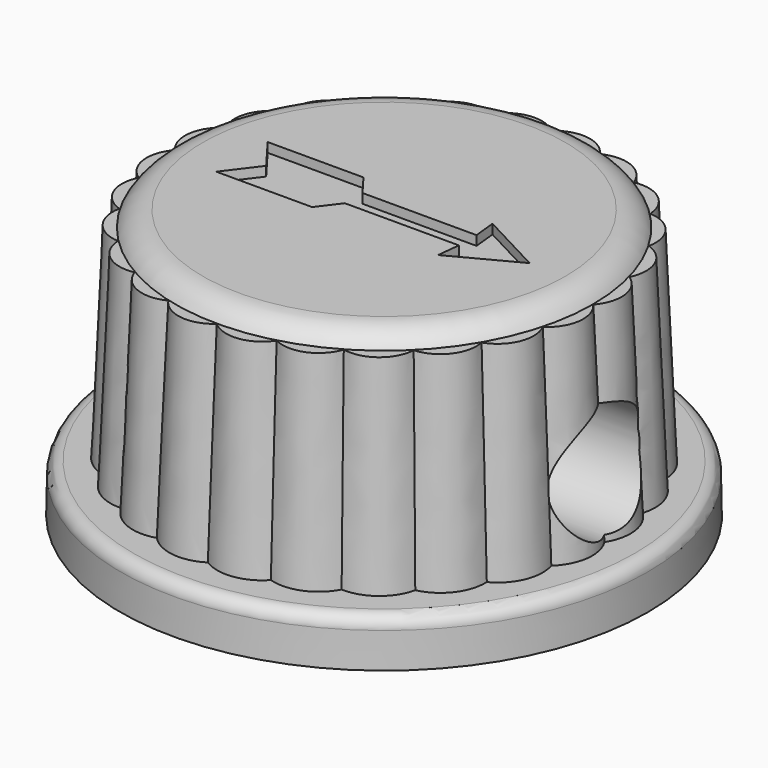
from build123d import *

# Parameters (mm, degrees)
F0_R                   = 8.35
F1_DEPTH               = 1.5
F1_TAPER               = 1
F2_R                   = 6.9
F3_DEPTH               = 6.5
F3_TAPER               = 2.5
F4_R                   = 6.6019829431
F5_DEPTH               = 0.5
F7_DEPTH               = 6.5
DRAFT_F7_DRAFTED_ANGLE = -2.5
F9_R                   = 0.4
F10_R                  = 3.9
F11_DEPTH              = 6.8
F12_R                  = 1.8
F13_DEPTH              = 25
F15_DEPTH              = 0.3


# Not quite as in the source:
# - a fillet or chamfer that OpenCascade refuses, or shapes differently, is made with other operations: its cross-section is extruded or revolved along the edge and cut away or added
# - an extrude with a draft is written as a straight extrude whose walls are then drafted


with BuildPart() as f1:
    # F0 (on Top) → F1 (new body)
    with BuildSketch(Plane.XY):
        Circle(F0_R)
    extrude(amount=F1_DEPTH, taper=F1_TAPER)

    # F2 (on face) → F3 (join)
    with BuildSketch(Plane.XY.offset(1.5)):
        Circle(F2_R)
    extrude(amount=F3_DEPTH, taper=F3_TAPER)

    # F4 (on face) → F5 (join)
    with BuildSketch(Plane.XY.offset(8)):
        Circle(F4_R)
    extrude(amount=F5_DEPTH)


with BuildPart() as f7_drafted:
    # F6 (on face) → F7 (new body, through all)
    with BuildSketch(Plane.XY.offset(8)):
        with BuildLine():
            ThreePointArc((6.3907621911, -1.7123995681), (6.8957390773, -0.9078412722), (6.6162038711, 0))
            ThreePointArc((6.6162038711, 0), (6.8957390773, 0.9078412722), (6.3907621911, 1.7123995681))
            ThreePointArc((6.3907621911, 1.7123995681), (6.4258058549, 2.6616559343), (5.729800629, 3.3081019355))
            ThreePointArc((5.729800629, 3.3081019355), (5.5179645827, 4.234083143), (4.678362623, 4.678362623))
            ThreePointArc((4.678362623, 4.678362623), (4.234083143, 5.5179645827), (3.3081019355, 5.729800629))
            ThreePointArc((3.3081019355, 5.729800629), (2.6616559343, 6.4258058549), (1.7123995681, 6.3907621911))
            ThreePointArc((1.7123995681, 6.3907621911), (0.9078412722, 6.8957390773), (0, 6.6162038711))
            ThreePointArc((0, 6.6162038711), (-0.9078412722, 6.8957390773), (-1.7123995681, 6.3907621911))
            ThreePointArc((-1.7123995681, 6.3907621911), (-2.6616559343, 6.4258058549), (-3.3081019355, 5.729800629))
            ThreePointArc((-3.3081019355, 5.729800629), (-4.234083143, 5.5179645827), (-4.678362623, 4.678362623))
            ThreePointArc((-4.678362623, 4.678362623), (-5.5179645827, 4.234083143), (-5.729800629, 3.3081019355))
            ThreePointArc((-5.729800629, 3.3081019355), (-6.4258058549, 2.6616559343), (-6.3907621911, 1.7123995681))
            ThreePointArc((-6.3907621911, 1.7123995681), (-6.8957390773, 0.9078412722), (-6.6162038711, 0))
            ThreePointArc((-6.6162038711, 0), (-6.8957390773, -0.9078412722), (-6.3907621911, -1.7123995681))
            ThreePointArc((-6.3907621911, -1.7123995681), (-6.4258058549, -2.6616559343), (-5.729800629, -3.3081019355))
            ThreePointArc((-5.729800629, -3.3081019355), (-5.5179645827, -4.234083143), (-4.678362623, -4.678362623))
            ThreePointArc((-4.678362623, -4.678362623), (-4.234083143, -5.5179645827), (-3.3081019355, -5.729800629))
            ThreePointArc((-3.3081019355, -5.729800629), (-2.6616559343, -6.4258058549), (-1.7123995681, -6.3907621911))
            ThreePointArc((-1.7123995681, -6.3907621911), (-0.9078412722, -6.8957390773), (0, -6.6162038711))
            ThreePointArc((0, -6.6162038711), (0.9078412722, -6.8957390773), (1.7123995681, -6.3907621911))
            ThreePointArc((1.7123995681, -6.3907621911), (2.6616559343, -6.4258058549), (3.3081019355, -5.729800629))
            ThreePointArc((3.3081019355, -5.729800629), (4.234083143, -5.5179645827), (4.678362623, -4.678362623))
            ThreePointArc((4.678362623, -4.678362623), (5.5179645827, -4.234083143), (5.729800629, -3.3081019355))
            ThreePointArc((5.729800629, -3.3081019355), (6.4258058549, -2.6616559343), (6.3907621911, -1.7123995681))
        make_face()
    extrude(amount=-F7_DEPTH)

    # draft_F7_drafted
    draft_f7_drafted_walls = [f7_drafted.faces().sort_by_distance(p)[0] for p in [
        (2.6616559343, -6.4258058549, 3.6666666667),
        (4.234083143, -5.5179645827, 3.6666666667),
        (5.5179645827, -4.234083143, 3.6666666667),
        (6.4258058549, -2.6616559343, 3.6666666667),
        (6.8957390773, -0.9078412722, 3.6666666667),
        (6.8957390773, 0.9078412722, 3.6666666667),
        (6.4258058549, 2.6616559343, 3.6666666667),
        (5.5179645827, 4.234083143, 3.6666666667),
        (4.234083143, 5.5179645827, 3.6666666667),
        (2.6616559343, 6.4258058549, 3.6666666667),
        (0.9078412722, 6.8957390773, 3.6666666667),
        (-0.9078412722, 6.8957390773, 3.6666666667),
        (-2.6616559343, 6.4258058549, 3.6666666667),
        (-4.234083143, 5.5179645827, 3.6666666667),
        (-5.5179645827, 4.234083143, 3.6666666667),
        (-6.4258058549, 2.6616559343, 3.6666666667),
        (-6.8957390773, 0.9078412722, 3.6666666667),
        (-6.8957390773, -0.9078412722, 3.6666666667),
        (-6.4258058549, -2.6616559343, 3.6666666667),
        (-5.5179645827, -4.234083143, 3.6666666667),
        (-4.234083143, -5.5179645827, 3.6666666667),
        (-2.6616559343, -6.4258058549, 3.6666666667),
        (-0.9078412722, -6.8957390773, 3.6666666667),
        (0.9078412722, -6.8957390773, 3.6666666667),
    ]]
    draft(draft_f7_drafted_walls, neutral_plane=Plane(origin=(0, 0, 8), x_dir=(1, 0, 0), z_dir=(0, 0, -1)), angle=DRAFT_F7_DRAFTED_ANGLE)


with BuildPart() as f1_1:
    add(f1.part)

    # join_F7_drafted: union F7_drafted
    add(f7_drafted.part)

    # F8: fillet of radius 1 on 1 edges, made by hand

    # F8_s1 → F8_t2 (revolve, cut)
    with BuildSketch(Plane.XZ):
        with BuildLine():
            ThreePointArc((6.6019829431, 8), (6.2359575393, 8.3660254038), (5.7359575393, 8.5))
            Line((5.7359575393, 8.5), (6.6019829431, 8.5))
            Line((6.6019829431, 8.5), (6.6019829431, 8))
        make_face()
    revolve(axis=Axis((0, 0, 8.5), (0, 0, 1)), mode=Mode.SUBTRACT)

    # F9
    f9_edges = [f1_1.edges().sort_by_distance(p)[0] for p in [
        (-8.323817, 0, 1.5),
    ]]
    fillet(f9_edges, radius=F9_R)

    # F10 (on face) → F11 (cut)
    with BuildSketch(Plane(origin=(0, 0, 0), x_dir=(1, 0, 0), z_dir=(0, 0, -1))):
        Circle(F10_R)
    extrude(amount=-F11_DEPTH, mode=Mode.SUBTRACT)

    # F12 (on Right) → F13 (cut)
    with BuildSketch(Plane.YZ):
        with Locations((0, 3.5)):
            Circle(F12_R)
    extrude(amount=F13_DEPTH, mode=Mode.SUBTRACT)

    # F14 (on face) → F15 (cut)
    with BuildSketch(Plane.XY.offset(8.5)):
        Polygon((-4.4968236719, 1.0159876547), (-3.7311276572, 0), (-4.4968236719, -1.0159876547), (-1.465461005, -1.0159876547), (-0.9635414288, -0.35), (2.6435573608, -0.35), (2.5679734536, -1.0748769855), (4.6023922041, 0), (2.5679734536, 1.0748769855), (2.6435573608, 0.35), (-0.9635414288, 0.35), (-1.465461005, 1.0159876547), align=None)
    extrude(amount=-F15_DEPTH, mode=Mode.SUBTRACT)


solid = f1_1.part
